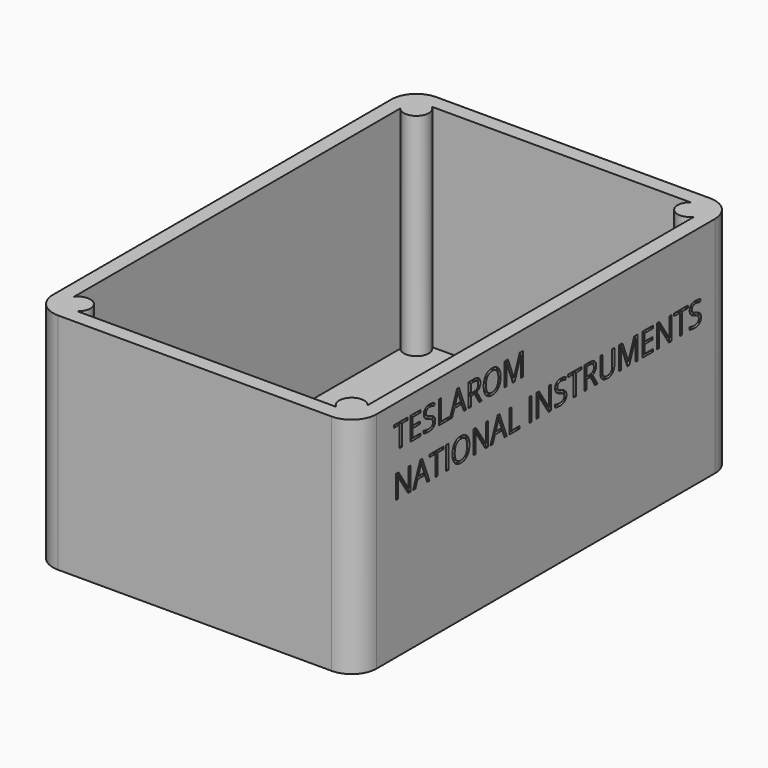
from build123d import *

# Parameters (mm, degrees)
F0_W         = 130
F0_H         = 190
F1_DEPTH     = 90
F2_R         = 10
F4_DEPTH     = 85
F5_TEXT_SIZE = 12.9631203082
F6_DEPTH     = 1


# Not quite as in the source:
# - Text() gives the source's letters only with a copy of the font that has no kerning and outlines rounded to 1/6400 em; it was checked with that copy


with BuildPart() as f1:
    # F0 (on Top) → F1 (new body)
    with BuildSketch(Plane.XY):
        with Locations((65, 95)):
            Rectangle(F0_W, F0_H)
    extrude(amount=F1_DEPTH)

    # F2
    f2_edges = [f1.edges().sort_by_distance(p)[0] for p in [
        (130, 0, 45),
        (130, 190, 45),
        (0, 0, 45),
        (0, 190, 45),
    ]]
    fillet(f2_edges, radius=F2_R)

    # F3 (on face) → F4 (cut)
    with BuildSketch(Plane.XY.offset(90)):
        with BuildLine():
            Line((117, 184), (13, 184))
            ThreePointArc((13, 184), (13.5355339059, 176.4644660941), (6, 177))
            Line((6, 177), (6, 13))
            ThreePointArc((6, 13), (13.5355339059, 13.5355339059), (13, 6))
            Line((13, 6), (117, 6))
            ThreePointArc((117, 6), (116.4644660941, 13.5355339059), (124, 13))
            Line((124, 13), (124, 177))
            ThreePointArc((124, 177), (116.4644660941, 176.4644660941), (117, 184))
        make_face()
    extrude(amount=-F4_DEPTH, mode=Mode.SUBTRACT)

    # F5 (on face) → F6 (cut)
    with BuildSketch(Plane.YZ.offset(130)):
        with Locations((18.5824334621, 73.2919946313)):
            Text('TESLAROM', F5_TEXT_SIZE, font='Open Sans', text_align=(TextAlign.LEFT, TextAlign.BOTTOM))
        with Locations((18.5824334621, 55.6621510122)):
            Text('NATIONAL INSTRUMENTS', F5_TEXT_SIZE, font='Open Sans', text_align=(TextAlign.LEFT, TextAlign.BOTTOM))
    extrude(amount=-F6_DEPTH, mode=Mode.SUBTRACT)


solid = f1.part
